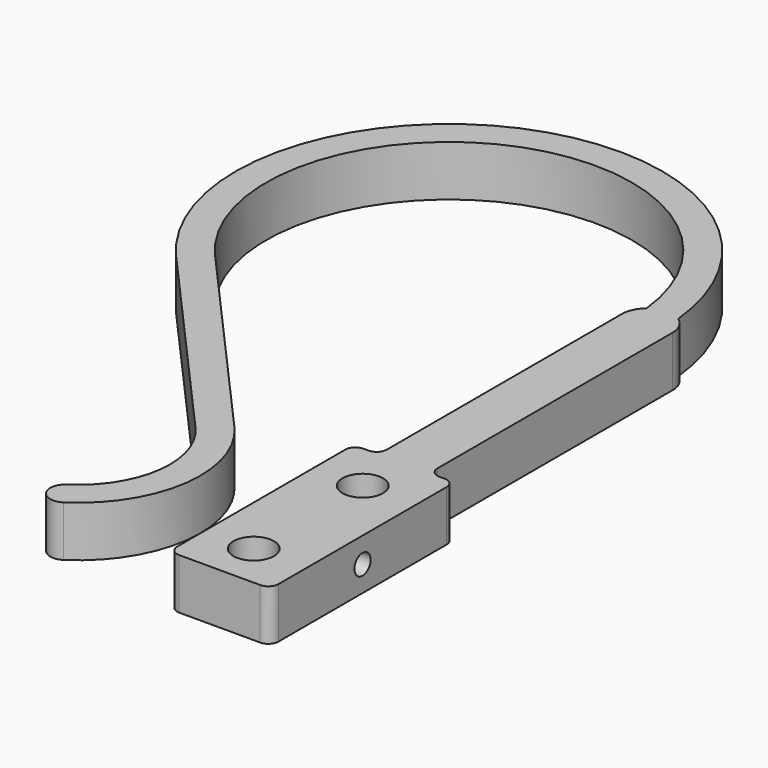
from build123d import *

# Parameters (mm, degrees)
F0_R     = 2
F1_DEPTH = 5
F2_R     = 1
F3_R     = 1
F4_DEPTH = 10


with BuildPart() as f1:
    # F0 (on Top) → F1 (new body)
    with BuildSketch(Plane.XY):
        Polygon((0, 22.7317288518), (0, 0), (10, 0), (10, 22.7317288518), (7.5, 22.7317288518), (5, 22.7317288518), (2.5, 22.7317288518), align=None)
        with Locations((4.8133912496, 4.4267121702)):
            Circle(F0_R, mode=Mode.SUBTRACT)
        with Locations((4.8133912496, 17.8769808263)):
            Circle(F0_R, mode=Mode.SUBTRACT)
        with BuildLine():
            Line((2.5, 52.7317288518), (2.5, 22.7317288518))
            Line((2.5, 22.7317288518), (5, 22.7317288518))
            Line((5, 22.7317288518), (5, 51.2317288518))
            ThreePointArc((5, 51.2317288518), (3.9393398282, 51.67106868), (3.5, 52.7317288518))
            ThreePointArc((3.5, 52.7317288518), (3.4744103207, 53.6926062484), (3.3977138284, 54.6507596031))
            ThreePointArc((3.3977138284, 54.6507596031), (2.7355226399, 53.7910410275), (2.5, 52.7317288518))
        make_face()
        with BuildLine():
            Line((5, 22.7317288518), (7.5, 22.7317288518))
            Line((7.5, 22.7317288518), (7.5, 52.7317288518))
            ThreePointArc((7.5, 52.7317288518), (7.2072929768, 53.9055506928), (6.3977138284, 54.8045038164))
            ThreePointArc((6.3977138284, 54.8045038164), (6.4744129083, 53.7693774574), (6.5, 52.7317288518))
            ThreePointArc((6.5, 52.7317288518), (6.0606601718, 51.67106868), (5, 51.2317288518))
            Line((5, 51.2317288518), (5, 22.7317288518))
        make_face()
        with BuildLine():
            ThreePointArc((3.5, 52.7317288518), (3.9393398282, 51.67106868), (5, 51.2317288518))
            Line((5, 51.2317288518), (5, 52.7317288518))
            ThreePointArc((5, 52.7317288518), (4.960003557, 53.9817288518), (4.8401778569, 55.226614998))
            ThreePointArc((4.8401778569, 55.226614998), (4.073091813, 55.053547366), (3.3977138284, 54.6507596031))
            ThreePointArc((3.3977138284, 54.6507596031), (3.4744103207, 53.6926062484), (3.5, 52.7317288518))
        make_face()
        with BuildLine():
            Line((5, 52.7317288518), (5, 51.2317288518))
            ThreePointArc((5, 51.2317288518), (6.0606601718, 51.67106868), (6.5, 52.7317288518))
            ThreePointArc((6.5, 52.7317288518), (6.4744129083, 53.7693774574), (6.3977138284, 54.8045038164))
            ThreePointArc((6.3977138284, 54.8045038164), (5.6539406843, 55.144685872), (4.8401778569, 55.226614998))
            ThreePointArc((4.8401778569, 55.226614998), (4.960003557, 53.9817288518), (5, 52.7317288518))
        make_face()
        with BuildLine():
            ThreePointArc((-28.0449956093, 40.7368995467), (-21.8583839955, 69.2405574995), (3.3977138284, 54.6507596031))
            ThreePointArc((3.3977138284, 54.6507596031), (4.073091813, 55.053547366), (4.8401778569, 55.226614998))
            ThreePointArc((4.8401778569, 55.226614998), (-21.968116408, 70.8241322208), (-30.1189319968, 40.8987017286))
            ThreePointArc((-30.1189319968, 40.8987017286), (-29.0493590182, 41.2357199074), (-28.0449956093, 40.7368995467))
        make_face()
        with BuildLine():
            ThreePointArc((4.8401778569, 55.226614998), (5.6539406843, 55.144685872), (6.3977138284, 54.8045038164))
            ThreePointArc((6.3977138284, 54.8045038164), (-22.9963973106, 72.0173965367), (-30.2870642065, 38.7436287659))
            ThreePointArc((-30.2870642065, 38.7436287659), (-30.661485659, 39.856935046), (-30.1189319968, 40.8987017286))
            ThreePointArc((-30.1189319968, 40.8987017286), (-21.968116408, 70.8241322208), (4.8401778569, 55.226614998))
        make_face()
        with BuildLine():
            Line((-9.0393445759, 19.3589845332), (-28.0449956093, 40.7368995467))
            ThreePointArc((-28.0449956093, 40.7368995467), (-27.6686113105, 39.6523008448), (-28.1693945175, 38.6192298577))
            Line((-28.1693945175, 38.6192298577), (-11.1570142649, 19.4833834414))
            ThreePointArc((-11.1570142649, 19.4833834414), (-10.0724155629, 19.8597677402), (-9.0393445759, 19.3589845332))
        make_face()
        with BuildLine():
            ThreePointArc((-28.1693945175, 38.6192298577), (-27.6686113105, 39.6523008448), (-28.0449956093, 40.7368995467))
            ThreePointArc((-28.0449956093, 40.7368995467), (-29.0493590182, 41.2357199074), (-30.1189319968, 40.8987017286))
            ThreePointArc((-30.1189319968, 40.8987017286), (-29.6535936799, 40.3103418877), (-29.1660299079, 39.7402641563))
            Line((-29.1660299079, 39.7402641563), (-28.1693945175, 38.6192298577))
        make_face()
        with BuildLine():
            ThreePointArc((-30.1189319968, 40.8987017286), (-30.661485659, 39.856935046), (-30.2870642065, 38.7436287659))
            ThreePointArc((-30.2870642065, 38.7436287659), (-29.2539932195, 38.2428455589), (-28.1693945175, 38.6192298577))
            Line((-28.1693945175, 38.6192298577), (-29.1660299079, 39.7402641563))
            ThreePointArc((-29.1660299079, 39.7402641563), (-29.6535936799, 40.3103418877), (-30.1189319968, 40.8987017286))
        make_face()
        with BuildLine():
            ThreePointArc((-28.1693945175, 38.6192298577), (-29.2539932195, 38.2428455589), (-30.2870642065, 38.7436287659))
            Line((-30.2870642065, 38.7436287659), (-11.2814131731, 17.3657137524))
            ThreePointArc((-11.2814131731, 17.3657137524), (-11.6577974719, 18.4503124544), (-11.1570142649, 19.4833834414))
            Line((-11.1570142649, 19.4833834414), (-28.1693945175, 38.6192298577))
        make_face()
        with BuildLine():
            ThreePointArc((-11.4373132839, 1.3031069234), (-6.1047109197, 9.7820673373), (-9.0393445759, 19.3589845332))
            ThreePointArc((-9.0393445759, 19.3589845332), (-8.6670458513, 18.2210817301), (-9.2461191516, 17.1731775156))
            ThreePointArc((-9.2461191516, 17.1731775156), (-10.3016462873, 16.8690161197), (-11.2814131731, 17.3657137524))
            ThreePointArc((-11.2814131731, 17.3657137524), (-9.0785988115, 10.1770240522), (-13.0813924983, 3.8124900222))
            ThreePointArc((-13.0813924983, 3.8124900222), (-13.5140444405, 1.7357588655), (-11.4373132839, 1.3031069234))
        make_face()
        with BuildLine():
            ThreePointArc((-9.2461191516, 17.1731775156), (-8.6670458513, 18.2210817301), (-9.0393445759, 19.3589845332))
            ThreePointArc((-9.0393445759, 19.3589845332), (-10.0724155629, 19.8597677402), (-11.1570142649, 19.4833834414))
            Line((-11.1570142649, 19.4833834414), (-10.1603788745, 18.3623491428))
            ThreePointArc((-10.1603788745, 18.3623491428), (-9.6820476982, 17.7840633382), (-9.2461191516, 17.1731775156))
        make_face()
        with BuildLine():
            ThreePointArc((-11.1570142649, 19.4833834414), (-11.6577974719, 18.4503124544), (-11.2814131731, 17.3657137524))
            ThreePointArc((-11.2814131731, 17.3657137524), (-10.3016462873, 16.8690161197), (-9.2461191516, 17.1731775156))
            ThreePointArc((-9.2461191516, 17.1731775156), (-9.6820476982, 17.7840633382), (-10.1603788745, 18.3623491428))
            Line((-10.1603788745, 18.3623491428), (-11.1570142649, 19.4833834414))
        make_face()
    extrude(amount=F1_DEPTH)

    # F2
    f2_edges = [f1.edges().sort_by_distance(p)[0] for p in [
        (0, 22.731729, 2.5),
        (2.5, 22.731729, 2.5),
        (10, 22.731729, 2.5),
        (7.5, 22.731729, 2.5),
        (10, 0, 2.5),
        (0, 0, 2.5),
    ]]
    fillet(f2_edges, radius=F2_R)

    # F3 (on face) → F4 (cut, through all)
    with BuildSketch(Plane.YZ.offset(10)):
        with Locations((11.3658644259, 2.5)):
            Circle(F3_R)
    extrude(amount=-F4_DEPTH, mode=Mode.SUBTRACT)


solid = f1.part
